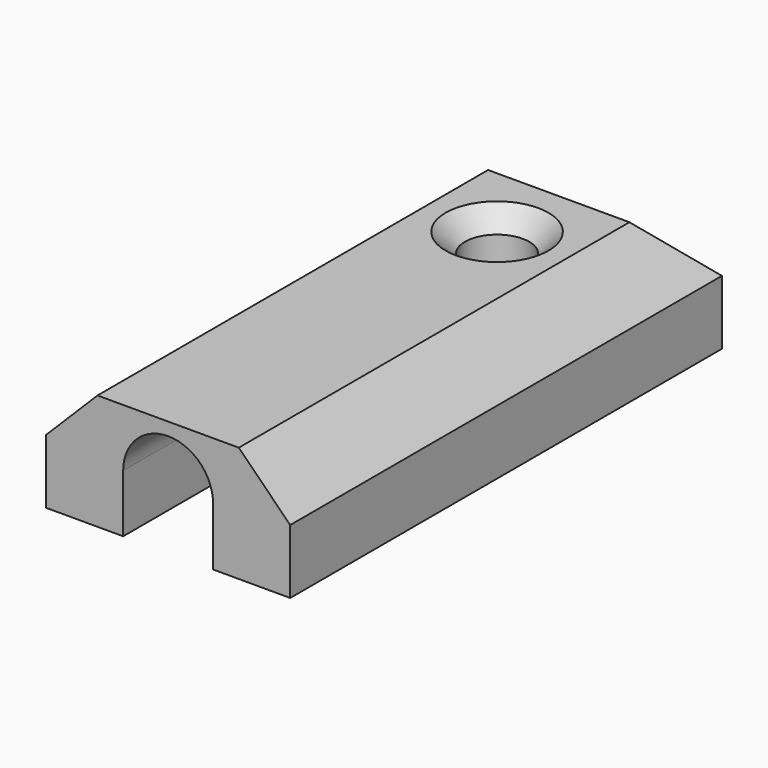
from build123d import *

# Parameters (mm, degrees)
F6_DEPTH        = 21
F7_SIZE         = 2
F8_SIZE         = 2
F12_DEPTH       = 2.251
F14_D           = 2.5
F14_CSINK_D     = 4
F14_CSINK_ANGLE = 90


# Not quite as in the source:
# - a feature names something its author has since deleted; it is built from what else it names


with BuildPart() as f6:
    # F5 (on Front) → F6 (new body)
    with BuildSketch(Plane.XZ):
        with BuildLine():
            Line((4.75, 0), (4.75, 4.5))
            Line((4.75, 4.5), (-4.75, 4.5))
            Line((-4.75, 4.5), (-4.75, 0))
            Line((-4.75, 0), (-1.75, 0))
            Line((-1.75, 0), (-1.75, 2.25))
            ThreePointArc((-1.75, 2.25), (0, 4), (1.75, 2.25))
            Line((1.75, 2.25), (1.75, 0))
            Line((1.75, 0), (4.75, 0))
        make_face()
        with BuildLine():
            Line((-1.75, 0), (1.75, 0))
            Line((1.75, 0), (1.75, 2.25))
            ThreePointArc((1.75, 2.25), (0, 4), (-1.75, 2.25))
            Line((-1.75, 2.25), (-1.75, 0))
        make_face()
    extrude(amount=-F6_DEPTH)

    # F7
    f7_edges = [f6.edges().sort_by_distance(p)[0] for p in [
        (-4.75, 10.5, 4.5),
        (4.75, 10.5, 4.5),
    ]]
    chamfer(f7_edges, length=F7_SIZE)

    # F8
    f8_edges = [f6.edges().sort_by_distance(p)[0] for p in [
        (0, 21, 4.5),
    ]]
    chamfer(f8_edges, length=F8_SIZE)

    # F10 (on offset) → F11 (revolve, cut)
    with BuildSketch(Plane.XY.offset(2.25)):
        with BuildLine():
            Line((-1.75, 11.75), (-1.75, 0))
            Line((-1.75, 0), (0, 0))
            Line((0, 0), (0, 13.5))
            ThreePointArc((0, 13.5), (-1.2374368671, 12.9874368671), (-1.75, 11.75))
        make_face()
    revolve(axis=Axis((0, 6.75, 2.25), (0, 1, 0)), mode=Mode.SUBTRACT)

    # F10 (on offset) → F12 (cut, through all)
    with BuildSketch(Plane.XY.offset(2.25)):
        with BuildLine():
            Line((-1.75, 11.75), (-1.75, 0))
            Line((-1.75, 0), (0, 0))
            Line((0, 0), (0, 13.5))
            ThreePointArc((0, 13.5), (-1.2374368671, 12.9874368671), (-1.75, 11.75))
        make_face()
        with BuildLine():
            Line((0, 13.5), (0, 0))
            Line((0, 0), (1.75, 0))
            Line((1.75, 0), (1.75, 11.75))
            ThreePointArc((1.75, 11.75), (1.2374368671, 12.9874368671), (0, 13.5))
        make_face()
    extrude(amount=-F12_DEPTH, mode=Mode.SUBTRACT)

    # F14 (through all)
    with Locations(Plane.XY.offset(4.5)):
        with Locations((0, 16)):
            CounterSinkHole(F14_D / 2, F14_CSINK_D / 2, counter_sink_angle=F14_CSINK_ANGLE)


solid = f6.part
